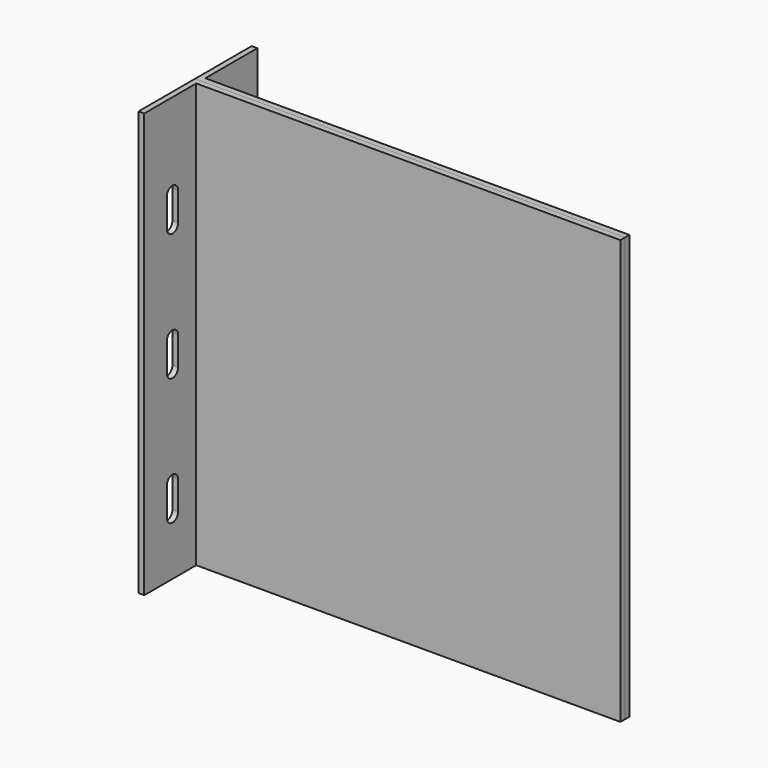
from build123d import *

# Parameters (mm, degrees)
F0_W     = 300
F0_H     = 300
F1_DEPTH = 4
F2_W     = 50
F2_H     = 300
F3_DEPTH = 4
F5_DEPTH = 25


# Not quite as in the source:
# - the program builds the solid bodies; features that only make, move or delete a surface that nothing else refers to are left out


with BuildPart() as f1:
    # F0 (on Front) → F1 (new body)
    with BuildSketch(Plane.XZ):
        with Locations((150, -150)):
            Rectangle(F0_W, F0_H)
    extrude(amount=F1_DEPTH)

    # F2 (on Right) → F3 (join)
    with BuildSketch(Plane.YZ):
        with Locations((-25, -150)):
            Rectangle(F2_W, F2_H)
    extrude(amount=-F3_DEPTH)

    # F4 (on face) → F5 (cut)
    with BuildSketch(Plane.YZ):
        with BuildLine():
            Line((-20, -80), (-20, -60))
            ThreePointArc((-20, -60), (-25, -55), (-30, -60))
            Line((-30, -60), (-30, -80))
            ThreePointArc((-30, -80), (-25, -85), (-20, -80))
        make_face()
        with BuildLine():
            Line((-20, -170), (-20, -150))
            ThreePointArc((-20, -150), (-25, -145), (-30, -150))
            Line((-30, -150), (-30, -170))
            ThreePointArc((-30, -170), (-25, -175), (-20, -170))
        make_face()
        with BuildLine():
            Line((-20, -260), (-20, -240))
            ThreePointArc((-20, -240), (-25, -235), (-30, -240))
            Line((-30, -240), (-30, -260))
            ThreePointArc((-30, -260), (-25, -265), (-20, -260))
        make_face()
    extrude(amount=-F5_DEPTH, mode=Mode.SUBTRACT)


with BuildPart() as f8_1:
    # F8: instance of F1
    add(f1.part.mirror(Plane.XZ))


solid = Compound([f1.part, f8_1.part])
